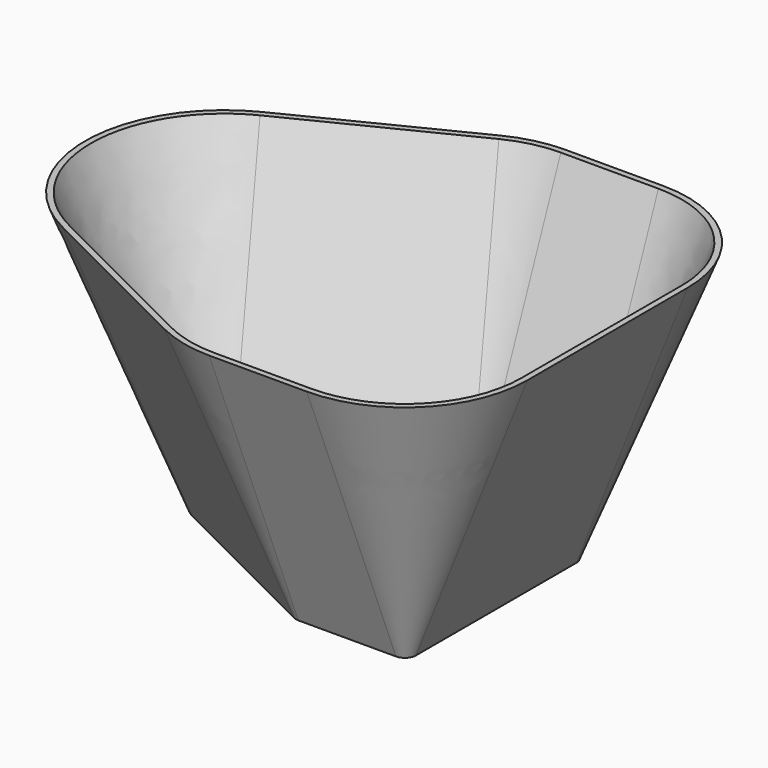
from build123d import *

# Parameters (mm, degrees)
F4_T = -1


with BuildPart() as f3:
    # F0 (on Top) → F3 section 0
    with BuildSketch(Plane.XY):
        with BuildLine():
            Line((-7.93628, 0.320123), (-25.464144, 0.320123))
            ThreePointArc((-25.464144, 0.320123), (-25.92365, 0.266621), (-26.358571, 0.108978))
            Line((-26.358571, 0.108978), (-56.992008, -15.207741))
            ThreePointArc((-56.992008, -15.207741), (-59.75594, -19.679877), (-56.992008, -24.152013))
            Line((-56.992008, -24.152013), (-26.358571, -39.468731))
            ThreePointArc((-26.358571, -39.468731), (-25.92365, -39.626375), (-25.464144, -39.679877))
            Line((-25.464144, -39.679877), (-7.93628, -39.679877))
            ThreePointArc((-7.93628, -39.679877), (-6.522066, -39.09409), (-5.93628, -37.679877))
            Line((-5.93628, -37.679877), (-5.93628, -1.679877))
            ThreePointArc((-5.93628, -1.679877), (-6.522066, -0.265663), (-7.93628, 0.320123))
        make_face()
    # F2 (on offset) → F3 section 1
    with BuildSketch(Plane.XY.offset(50)):
        with BuildLine():
            Line((-7.93628, 20.320123), (-25.464144, 20.320123))
            ThreePointArc((-25.464144, 20.320123), (-30.518708, 19.731601), (-35.302843, 17.997521))
            Line((-35.302843, 17.997521), (-65.93628, 2.680803))
            ThreePointArc((-65.93628, 2.680803), (-79.75594, -19.679877), (-65.93628, -42.040557))
            Line((-65.93628, -42.040557), (-35.302843, -57.357275))
            ThreePointArc((-35.302843, -57.357275), (-30.518708, -59.091355), (-25.464144, -59.679877))
            Line((-25.464144, -59.679877), (-7.93628, -59.679877))
            ThreePointArc((-7.93628, -59.679877), (7.62007, -53.236226), (14.06372, -37.679877))
            Line((14.06372, -37.679877), (14.06372, -1.679877))
            ThreePointArc((14.06372, -1.679877), (7.62007, 13.876472), (-7.93628, 20.320123))
        make_face()
    loft()

    # F4
    f4_openings = [f3.faces().sort_by_distance(p)[0] for p in [
        (-27.581923, -19.679877, 50),
    ]]
    offset(amount=F4_T, openings=f4_openings)


solid = f3.part
